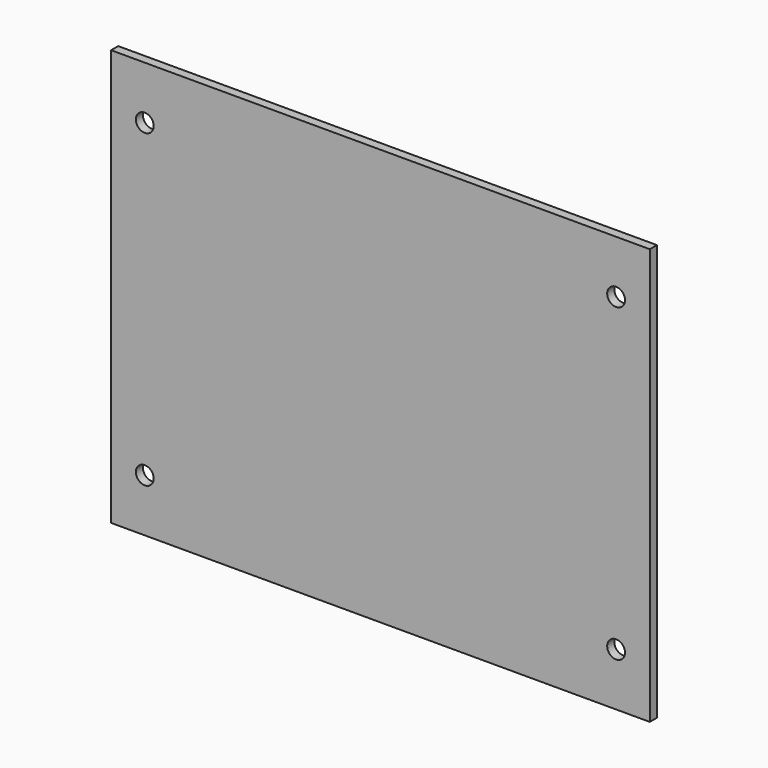
from build123d import *

# Parameters (mm, degrees)
F1_W     = 3.807
F1_H     = 2.9409
F1_R     = 0.0629689606
F1_R_2   = 0.0630157123
F1_R_3   = 0.0630453805
F2_DEPTH = 0.063
F3_SCALE = 25.4


with BuildPart() as f2:
    # F1 (on Front) → F2 (new body)
    with BuildSketch(Plane.XZ):
        Rectangle(F1_W, F1_H)
        with Locations((-1.6654, -1.09645)):
            Circle(F1_R, mode=Mode.SUBTRACT)
        with Locations((1.6654, -1.09645)):
            Circle(F1_R_2, mode=Mode.SUBTRACT)
        with Locations((-1.6654, 1.09645)):
            Circle(F1_R_3, mode=Mode.SUBTRACT)
        with Locations((1.6654, 1.09645)):
            Circle(F1_R_2, mode=Mode.SUBTRACT)
    extrude(amount=F2_DEPTH)


with BuildPart() as f2_1:
    # F3: moved
    add(f2.part.scale(F3_SCALE).moved(Location((-46.4454, 1.5372, 35.87898))))


solid = f2_1.part
